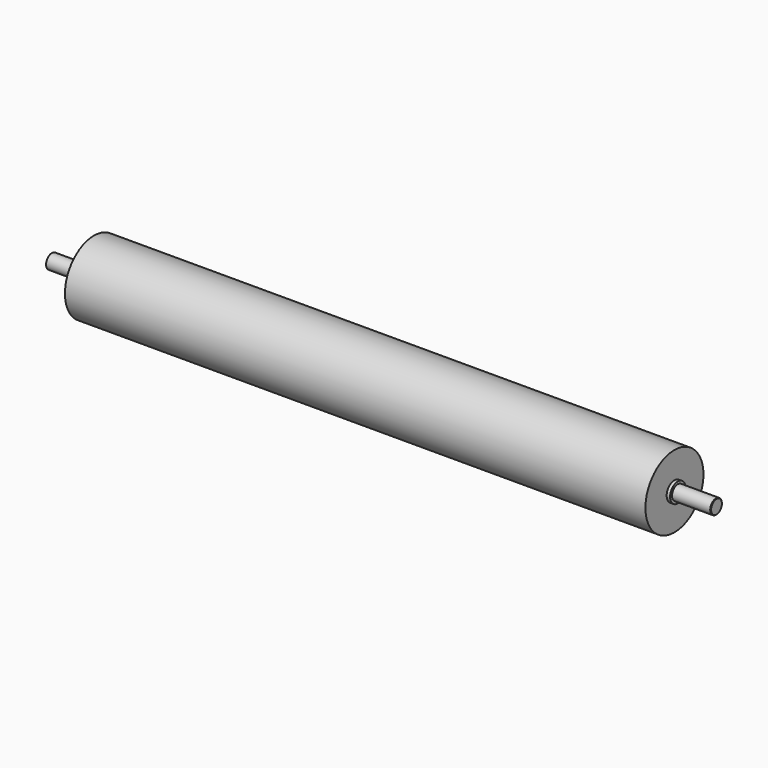
from build123d import *

# Parameters (mm, degrees)
F0_R      = 75
F1_DEPTH  = 600
F2_R      = 20
F3_DEPTH  = 150
F4_R      = 20
F5_DEPTH  = 150
F6_W      = 4.2212159717
F6_H      = 12
F7_DEPTH  = 125
F8_R      = 20
F9_DEPTH  = 157
F10_R     = 15
F11_DEPTH = 80
F14_DEPTH = 8.8
F16_R     = 30
F17_DEPTH = 25
F18_DEPTH = 92
F19_SIZE  = 1


with BuildPart() as f1:
    # F0 (on Right) → F1 (new body, symmetric)
    with BuildSketch(Plane.YZ):
        Circle(F0_R)
    extrude(amount=F1_DEPTH, both=True)

    # F2 (on face) → F3 (cut)
    with BuildSketch(Plane.YZ.offset(600)):
        Circle(F2_R)
    extrude(amount=-F3_DEPTH, mode=Mode.SUBTRACT)

    # F4 (on face) → F5 (cut)
    with BuildSketch(Plane(origin=(-600, 0, 0), x_dir=(0, -1, 0), z_dir=(-1, 0, 0))):
        Circle(F4_R)
    extrude(amount=-F5_DEPTH, mode=Mode.SUBTRACT)

    # F6 (on face) → F7 (cut)
    with BuildSketch(Plane.YZ.offset(600)):
        with Locations((21.1893920142, 0)):
            Rectangle(F6_W, F6_H)
    extrude(amount=-F7_DEPTH, mode=Mode.SUBTRACT)


with BuildPart() as f9:
    # F8 (on face) → F9 (new body)
    with BuildSketch(Plane.YZ.offset(450)):
        Circle(F8_R)
    extrude(amount=F9_DEPTH)

    # F10 (on face) → F11 (join)
    with BuildSketch(Plane.YZ.offset(607)):
        Circle(F10_R)
    extrude(amount=F11_DEPTH)


with BuildPart() as f12_1:
    # F12: instance of F9
    add(f9.part.mirror(Plane.YZ))

    # F18 (add): a face of the model
    f18_faces = [f12_1.faces().sort_by_distance(p)[0] for p in [
        (-687, 0, 0),
    ]]
    extrude(f18_faces, amount=-F18_DEPTH)


with BuildPart() as f14_tool:
    # F13 (on face) → F14 (new body)
    with BuildSketch(Plane.XZ.offset(-23.3)):
        with BuildLine():
            ThreePointArc((475, 6), (469, 0), (475, -6))
            Line((475, -6), (575, -6))
            ThreePointArc((575, -6), (581, 0), (575, 6))
            Line((575, 6), (475, 6))
        make_face()
    extrude(amount=F14_DEPTH)


with BuildPart() as f1_1:
    add(f1.part)

    # F14: cut by f14_tool
    add(f14_tool.part, mode=Mode.SUBTRACT)

    # F16 (on offset) → F17 (cut)
    with BuildSketch(Plane.YZ.offset(475)):
        Circle(F16_R)
    extrude(amount=-F17_DEPTH, mode=Mode.SUBTRACT)


with BuildPart() as f9_1:
    add(f9.part)

    # F14: cut by f14_tool
    add(f14_tool.part, mode=Mode.SUBTRACT)

    # F19
    f19_edges = [f9_1.edges().sort_by_distance(p)[0] for p in [
        (687, -15, 0),
    ]]
    chamfer(f19_edges, length=F19_SIZE)


solid = Compound([f12_1.part, f1_1.part, f9_1.part])
